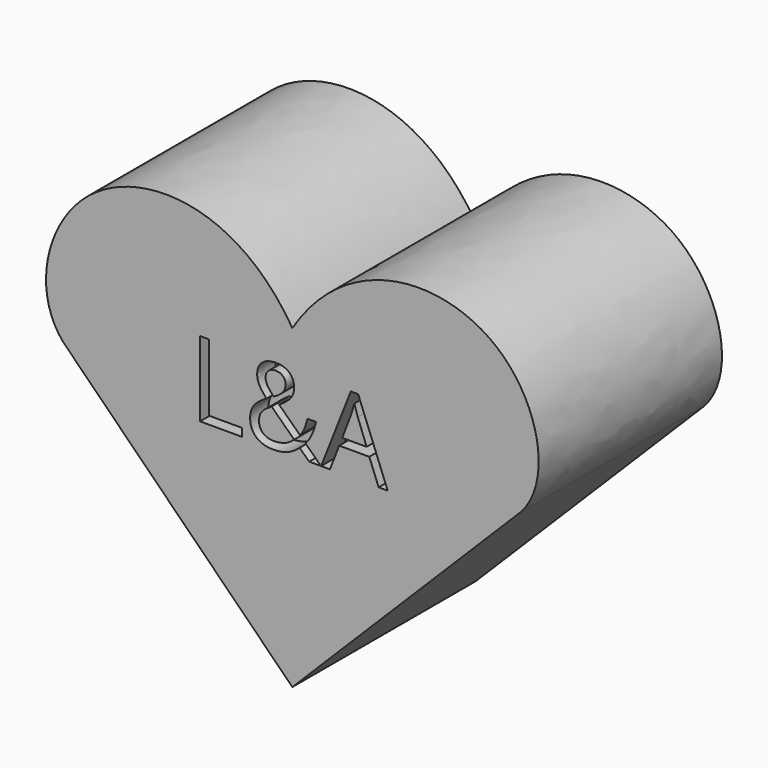
from build123d import *

# Parameters (mm, degrees)
F1_DEPTH     = 50.8
F2_TEXT_SIZE = 23.3211658067
F3_DEPTH     = 5.08


# Not quite as in the source:
# - Text() gives the source's letters only with a copy of the font that has no kerning and outlines rounded to 1/6400 em; it was checked with that copy


with BuildPart() as f1:
    # F0 (on Front) → F1 (new body)
    with BuildSketch(Plane.XZ):
        with BuildLine():
            Line((-50.8, 50.8), (0, 0))
            Line((0, 0), (50.8, 50.8))
            add(Edge.make_bspline(
                [(50.8, 50.8), (57.7898084712, 58.7500814685), (50.9510941858, 91.4292289752), (12.2052401163, 89.8069547992), (0, 70.032171905)],
                knots=[0, 0, 0, 0, 0.4488147171, 1, 1, 1, 1], degree=3))
            add(Edge.make_bspline(
                [(-50.8, 50.8), (-57.7898084712, 58.7500814685), (-50.9510941858, 91.4292289752), (-12.2052401163, 89.8069547992), (0, 70.032171905)],
                knots=[0, 0, 0, 0, 0.4488147171, 1, 1, 1, 1], degree=3))
        make_face()
    extrude(amount=F1_DEPTH)

    # F2 (on face) → F3 (cut)
    with BuildSketch(Plane.XZ.offset(50.8)):
        with Locations((-22.752130666, 45.2112443745)):
            Text('L&A', F2_TEXT_SIZE, font='Open Sans', text_align=(TextAlign.LEFT, TextAlign.BOTTOM))
    extrude(amount=-F3_DEPTH, mode=Mode.SUBTRACT)


solid = f1.part
